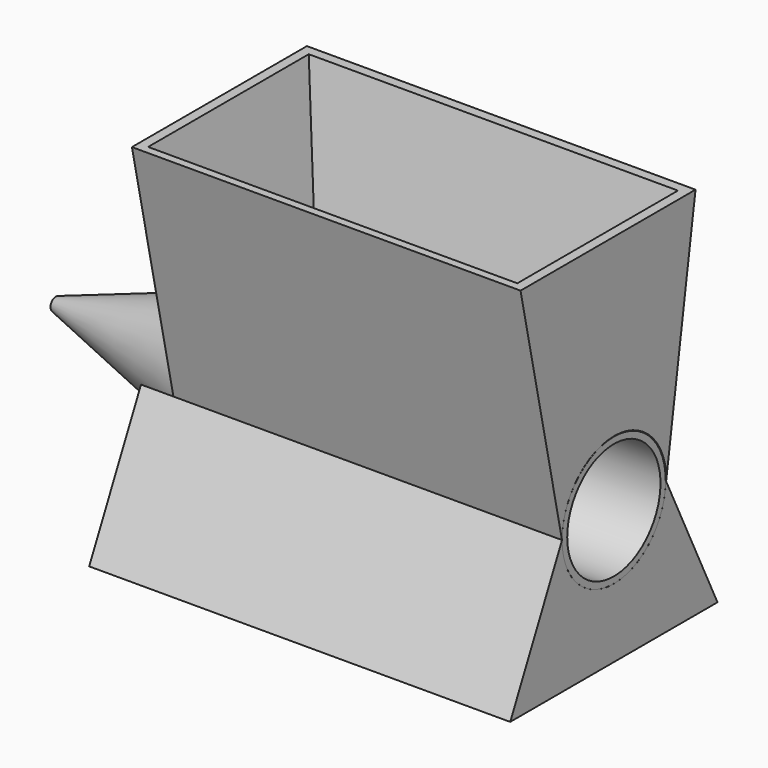
from build123d import *

# Parameters (mm, degrees)
F0_W      = 60
F0_H      = 10
F2_R      = 9
F3_DEPTH  = 60
F7_DEPTH  = 60
F8_W      = 57
F8_H      = 31
F9_DEPTH  = 37
F9_TAPER  = 12
F11_DEPTH = 65


# Not quite as in the source:
# - ends of sketch curves that miss each other by under 0.0002 mm in the source are joined


with BuildPart() as f1:
    # F0 (on Front) → F1 (revolve)
    with BuildSketch(Plane.XZ):
        with Locations((2.5320472605, 5)):
            Rectangle(F0_W, F0_H)
    revolve(axis=Axis((2.5320472605, 0, 0), (1, 0, 0)))

    # F2 (on face) → F3 (cut)
    with BuildSketch(Plane(origin=(-27.4679527395, 0, 0), x_dir=(0, -1, 0), z_dir=(-1, 0, 0))):
        Circle(F2_R)
    extrude(amount=-F3_DEPTH, mode=Mode.SUBTRACT)

    # F4 (on Front) → F5 (revolve)
    with BuildSketch(Plane.XZ):
        Polygon((-27.3532667905, 0), (-27.3532667905, 9.7150442334), (-53.6260029736, 1.0178652923), (-53.3532667905, 0), align=None)
    revolve(axis=Axis((2.5320472605, 0, 0), (1, 0, 0)))


with BuildPart() as f7:
    # F6 (on face) → F7 (new body)
    with BuildSketch(Plane.YZ.offset(32.5320472605)):
        with BuildLine():
            Line((-18.0040858686, 37.1578894556), (-10, 0))
            ThreePointArc((-10, 0), (0.0573891046, 10.0573938269), (10.1147829316, 0))
            Line((10.1147829316, 0), (15.7607458532, 37.1578894556))
            Line((15.7607458532, 37.1578894556), (-18.0040858686, 37.1578894556))
        make_face()
    extrude(amount=-F7_DEPTH)


with BuildPart() as f9_tool:
    # F8 (on face) → F9 (new body)
    with BuildSketch(Plane.XY.offset(37.1578894556)):
        with Locations((2.5320472605, -1.2540858686)):
            Rectangle(F8_W, F8_H)
    extrude(amount=-F9_DEPTH, taper=F9_TAPER)


with BuildPart() as f1_1:
    add(f1.part)

    # F9: cut by f9_tool
    add(f9_tool.part, mode=Mode.SUBTRACT)


with BuildPart() as f7_1:
    add(f7.part)

    # F9: cut by f9_tool
    add(f9_tool.part, mode=Mode.SUBTRACT)


with BuildPart() as f11:
    # F10 (on face) → F11 (new body)
    with BuildSketch(Plane.YZ.offset(32.5320472605)):
        with BuildLine():
            ThreePointArc((10, 0), (0, -10), (-10, 0))
            Line((-10, 0), (-20, -20.6474160484))
            Line((-20, -20.6474160484), (20, -20.6474160484))
            Line((20, -20.6474160484), (10, 0))
        make_face()
    extrude(amount=-F11_DEPTH)


solid = Compound([f1_1.part, f7_1.part, f11.part])
